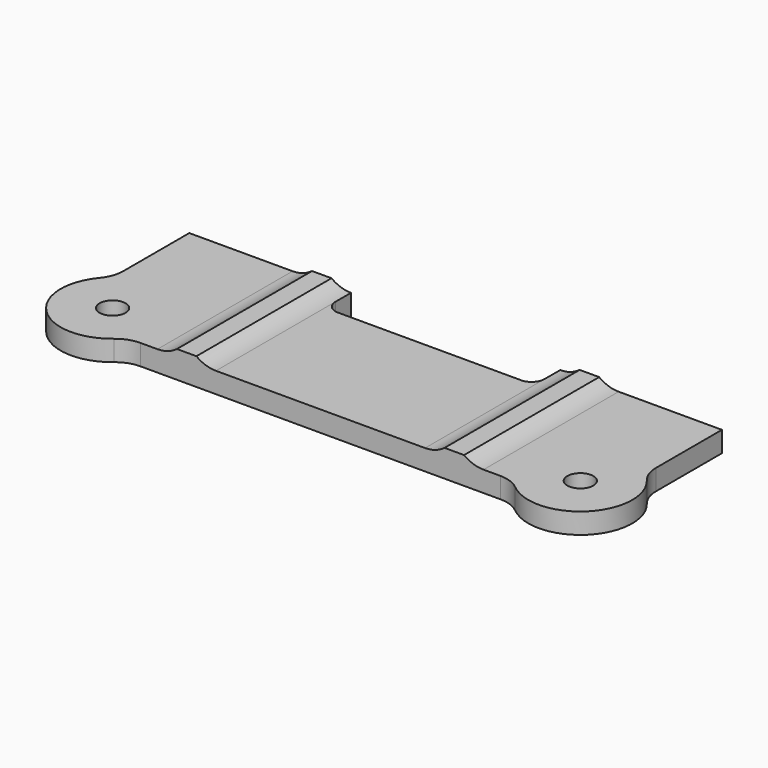
from build123d import *

# Parameters (mm, degrees)
F0_R        = 2
F1_DEPTH    = 3.175
F2_R        = 5
F3_R        = 2
F4_W        = 3
F4_H        = 26
F5_DEPTH    = 1
F6_T1_DEPTH = 26


# Not quite as in the source:
# - a fillet or chamfer that OpenCascade refuses, or shapes differently, is made with other operations: its cross-section is extruded or revolved along the edge and cut away or added


with BuildPart() as f1:
    # F0 (on Top) → F1 (new body)
    with BuildSketch(Plane.XY):
        with BuildLine():
            Line((11.2449979984, 0), (0, 0))
            Line((0, 0), (0, 11.2449979984))
            ThreePointArc((0, 11.2449979984), (-0.6568542495, -0.6568542495), (11.2449979984, 0))
        make_face()
        Polygon((0, 11.2449979984), (0, 0), (11.2449979984, 0), (41, 0), (70.7550020016, 0), (82, 0), (82, 11.2449979984), (82, 26), (57.1, 26), (57.1, 21), (41, 21), (24.9, 21), (24.9, 26), (0, 26), align=None)
        with Locations((5, 5)):
            Circle(F0_R, mode=Mode.SUBTRACT)
        with Locations((77, 5)):
            Circle(F0_R, mode=Mode.SUBTRACT)
        with BuildLine():
            Line((82, 0), (70.7550020016, 0))
            ThreePointArc((70.7550020016, 0), (82.6568542495, -0.6568542495), (82, 11.2449979984))
            Line((82, 11.2449979984), (82, 0))
        make_face()
    extrude(amount=F1_DEPTH)

    # F2
    f2_edges = [f1.edges().sort_by_distance(p)[0] for p in [
        (11.244998, 0, 1.5875),
        (70.755002, 0, 1.5875),
        (82, 11.244998, 1.5875),
        (0, 11.244998, 1.5875),
    ]]
    fillet(f2_edges, radius=F2_R)

    # F3
    f3_edges = [f1.edges().sort_by_distance(p)[0] for p in [
        (24.9, 21, 1.5875),
        (57.1, 21, 1.5875),
    ]]
    fillet(f3_edges, radius=F3_R)

    # F4 (on face) → F5 (join)
    with BuildSketch(Plane.XY.offset(3.175)):
        with Locations((20.4, 13)):
            Rectangle(F4_W, F4_H)
        with Locations((61.6, 13)):
            Rectangle(F4_W, F4_H)
    extrude(amount=F5_DEPTH)

    # F6: fillet of radius 5 on 4 edges, made by hand

    # F6_s2 → F6_t1 (join)
    with BuildSketch(Plane.XZ.offset(-26)):
        with BuildLine():
            ThreePointArc((15.9, 3.175), (17.4811388301, 3.4315835097), (18.9, 4.175))
            Line((18.9, 4.175), (18.96, 4.095))
            ThreePointArc((18.96, 4.095), (19, 3.675), (19, 3.175))
            Line((19, 3.175), (18.9, 3.075))
            Line((18.9, 3.075), (15.9, 3.075))
            Line((15.9, 3.075), (15.9, 3.175))
        make_face()
        with BuildLine():
            ThreePointArc((24.9, 3.175), (23.3188611699, 3.4315835097), (21.9, 4.175))
            Line((21.9, 4.175), (21.84, 4.095))
            ThreePointArc((21.84, 4.095), (21.8, 3.675), (21.8, 3.175))
            Line((21.8, 3.175), (21.9, 3.075))
            Line((21.9, 3.075), (24.9, 3.075))
            Line((24.9, 3.075), (24.9, 3.175))
        make_face()
        with BuildLine():
            ThreePointArc((57.1, 3.175), (58.6811388301, 3.4315835097), (60.1, 4.175))
            Line((60.1, 4.175), (60.16, 4.095))
            ThreePointArc((60.16, 4.095), (60.2, 3.675), (60.2, 3.175))
            Line((60.2, 3.175), (60.1, 3.075))
            Line((60.1, 3.075), (57.1, 3.075))
            Line((57.1, 3.075), (57.1, 3.175))
        make_face()
        with BuildLine():
            ThreePointArc((66.1, 3.175), (64.5188611699, 3.4315835097), (63.1, 4.175))
            Line((63.1, 4.175), (63.04, 4.095))
            ThreePointArc((63.04, 4.095), (63, 3.675), (63, 3.175))
            Line((63, 3.175), (63.1, 3.075))
            Line((63.1, 3.075), (66.1, 3.075))
            Line((66.1, 3.075), (66.1, 3.175))
        make_face()
    extrude(amount=F6_T1_DEPTH)


solid = f1.part
